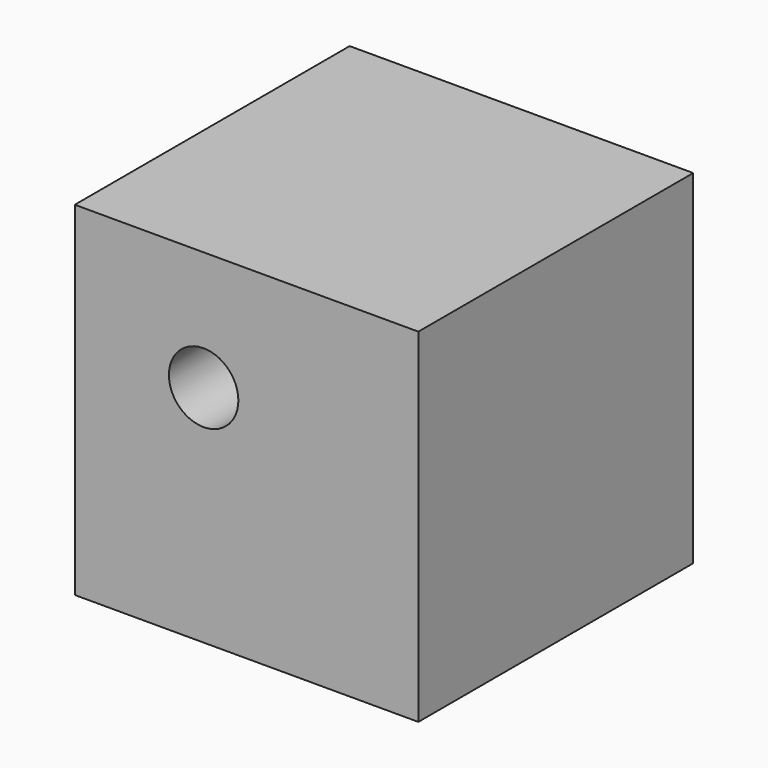
from build123d import *

# Parameters (mm, degrees)
F1_DEPTH = 76.2
F2_R     = 7.702083685
F3_DEPTH = 76.2


# Not quite as in the source:
# - a feature names something its author has since deleted; it is built from what else it names


with BuildPart() as f1:
    # F0 (on Front) → F1 (new body)
    with BuildSketch(Plane.XZ):
        Polygon((-37.524404479, 59.8273601898), (-37.524404479, -16.3726398102), (38.675595521, -16.3726398102), (38.675595521, 59.8273601898), (35.8841840983, 59.8273601898), align=None)
    extrude(amount=F1_DEPTH)

    # F2 (on face) → F3 (cut)
    with BuildSketch(Plane.XZ.offset(76.2)):
        with Locations((-8.9478027076, 33.3981923759)):
            Circle(F2_R)
    extrude(amount=-F3_DEPTH, mode=Mode.SUBTRACT)


solid = f1.part
